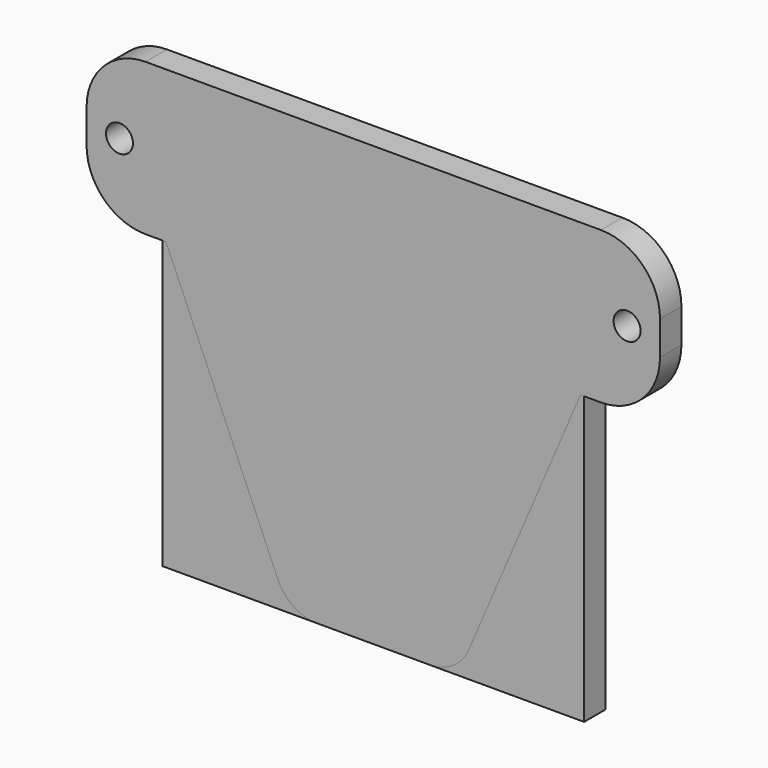
from build123d import *

# Parameters (mm, degrees)
F0_R        = 1.6
F1_DEPTH    = 3.175
F2_R        = 7
F4_T4_DEPTH = 184.6299677566
F4_T9_DEPTH = 184.6299677566
F5_R        = 5.08


# Not quite as in the source:
# - a fillet or chamfer that OpenCascade refuses, or shapes differently, is made with other operations: its cross-section is extruded or revolved along the edge and cut away or added


with BuildPart() as f1:
    # F0 (on Front) → F1 (new body)
    with BuildSketch(Plane.XZ):
        Polygon((-25, 13), (-25, -21), (25, -21), (25, 13), (34, 13), (34, 22), (34, 31), (0, 31), (-34, 31), (-34, 24), (-34, 13), align=None)
        with Locations((-30.099, 22)):
            Circle(F0_R, mode=Mode.SUBTRACT)
        with Locations((30.099, 22)):
            Circle(F0_R, mode=Mode.SUBTRACT)
    extrude(amount=F1_DEPTH)

    # F2
    f2_edges = [f1.edges().sort_by_distance(p)[0] for p in [
        (-34, -1.5875, 31),
        (-34, -1.5875, 13),
        (34, -1.5875, 31),
        (34, -1.5875, 13),
    ]]
    fillet(f2_edges, radius=F2_R)


with BuildPart() as f3_1:
    # F3: copy of F1
    add(f1.part)


with BuildPart() as f1_1:
    add(f1.part)

    # F4: chamfer of 15 x 35 on 2 edges, made by hand


with BuildPart() as f4_tool2:
    # F4_s3 → F4_t4 (new body)
    with BuildSketch(Plane.XZ.offset(-90.7274838783)):
        Polygon((-10, -21), (-25, 14), (-25, -21), align=None)
    extrude(amount=F4_T4_DEPTH)

    split(bisect_by=Plane.XY.offset(13), keep=Keep.BOTTOM)


with BuildPart() as f1_2:
    add(f1_1.part)

    # F4_t1: cut F4_tool2
    add(f4_tool2.part, mode=Mode.SUBTRACT)


with BuildPart() as f4_tool7:
    # F4_s8 → F4_t9 (new body)
    with BuildSketch(Plane.XZ.offset(-90.7274838783)):
        Polygon((25, 14), (10, -21), (25, -21), align=None)
    extrude(amount=F4_T9_DEPTH)

    split(bisect_by=Plane.XY.offset(13), keep=Keep.BOTTOM)


with BuildPart() as f1_3:
    add(f1_2.part)

    # F4_t6: cut F4_tool7
    add(f4_tool7.part, mode=Mode.SUBTRACT)

    # F5
    f5_edges = [f1_3.edges().sort_by_distance(p)[0] for p in [
        (-10, -1.5875, -21),
        (10, -1.5875, -21),
    ]]
    fillet(f5_edges, radius=F5_R)


solid = Compound([f3_1.part, f1_3.part])
